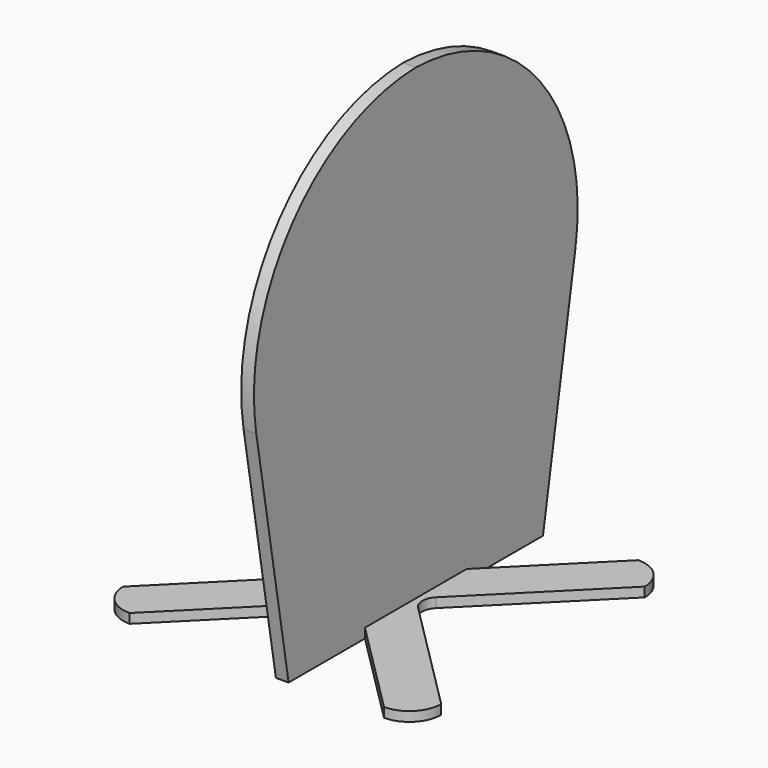
from build123d import *

# Parameters (mm, degrees)
F1_DEPTH    = 3
F2_R        = 9.99999
F3_R        = 5
F4_DEPTH    = 50
F6_DEPTH    = 10
F7_DEPTH    = 6
F8_T1_DEPTH = 387.2306894548
F9_R        = 9.99999
F10_R       = 5.99999


# Not quite as in the source:
# - a fillet or chamfer that OpenCascade refuses, or shapes differently, is made with other operations: its cross-section is extruded or revolved along the edge and cut away or added
# - a fillet or chamfer is up to 0.001 mm smaller than in the source, because OpenCascade refuses the exact size


with BuildPart() as f1:
    # F0 (on Top) → F1 (new body)
    with BuildSketch(Plane.XY):
        with BuildLine():
            Line((0, 10), (10, 0))
            ThreePointArc((10, 0), (7.0710678119, 7.0710678119), (0, 10))
        make_face()
        with BuildLine():
            Line((50, -40), (10, 0))
            ThreePointArc((10, 0), (7.0710678119, -7.0710678119), (0, -10))
            Line((0, -10), (40, -50))
            Line((40, -50), (50, -50))
            Line((50, -50), (50, -40))
        make_face()
        Polygon((0, -10), (10, 0), (0, 10), (-10, 0), align=None)
        with BuildLine():
            ThreePointArc((0, 10), (7.0710678119, 7.0710678119), (10, 0))
            Line((10, 0), (50, 40))
            Line((50, 40), (50, 50))
            Line((50, 50), (40, 50))
            Line((40, 50), (0, 10))
        make_face()
        with BuildLine():
            ThreePointArc((0, -10), (7.0710678119, -7.0710678119), (10, 0))
            Line((10, 0), (0, -10))
        make_face()
        with BuildLine():
            Line((-10, 0), (0, 10))
            ThreePointArc((0, 10), (-7.0710678119, 7.0710678119), (-10, 0))
        make_face()
        with BuildLine():
            ThreePointArc((-10, 0), (-7.0710678119, 7.0710678119), (0, 10))
            Line((0, 10), (-40, 50))
            Line((-40, 50), (-50, 50))
            Line((-50, 50), (-50, 40))
            Line((-50, 40), (-10, 0))
        make_face()
        with BuildLine():
            Line((-40, -50), (0, -10))
            ThreePointArc((0, -10), (-7.0710678119, -7.0710678119), (-10, 0))
            Line((-10, 0), (-50, -40))
            Line((-50, -40), (-50, -50))
            Line((-50, -50), (-40, -50))
        make_face()
        with BuildLine():
            ThreePointArc((-10, 0), (-7.0710678119, -7.0710678119), (0, -10))
            Line((0, -10), (-10, 0))
        make_face()
    extrude(amount=F1_DEPTH)

    # F2 (radius 10 in the source; OpenCascade refuses exactly that, so slightly less here)
    f2_edges = [f1.edges().sort_by_distance(p)[0] for p in [
        (-50, 50, 1.5),
        (-50, -50, 1.5),
        (50, -50, 1.5),
        (50, 50, 1.5),
    ]]
    fillet(f2_edges, radius=F2_R)

    # F3
    f3_edges = [f1.edges().sort_by_distance(p)[0] for p in [
        (10, 0, 1.5),
        (0, 10, 1.5),
        (-10, 0, 1.5),
        (0, -10, 1.5),
    ]]
    fillet(f3_edges, radius=F3_R)

    # F0 (on Top) → F4 (join)
    with BuildSketch(Plane.XY):
        with BuildLine():
            Line((0, 10), (10, 0))
            ThreePointArc((10, 0), (7.0710678119, 7.0710678119), (0, 10))
        make_face()
        Polygon((0, -10), (10, 0), (0, 10), (-10, 0), align=None)
        with BuildLine():
            ThreePointArc((0, -10), (7.0710678119, -7.0710678119), (10, 0))
            Line((10, 0), (0, -10))
        make_face()
        with BuildLine():
            Line((-10, 0), (0, 10))
            ThreePointArc((0, 10), (-7.0710678119, 7.0710678119), (-10, 0))
        make_face()
        with BuildLine():
            ThreePointArc((-10, 0), (-7.0710678119, -7.0710678119), (0, -10))
            Line((0, -10), (-10, 0))
        make_face()
    extrude(amount=F4_DEPTH)

    # F5 (on Right) → F6 (join)
    with BuildSketch(Plane.YZ):
        with BuildLine():
            Line((-70.7106781187, 120.7106781187), (0, 150))
            ThreePointArc((0, 150), (-37.3285426078, 146.4855717522), (-73.3452003698, 136.0657990677))
            Line((-73.3452003698, 136.0657990677), (-70.7106781187, 120.7106781187))
        make_face()
        Polygon((-64.6446609407, 85.3553390593), (0, 150), (-70.7106781187, 120.7106781187), align=None)
        Polygon((-50, 0), (0, 0), (0, 150), (-64.6446609407, 85.3553390593), align=None)
        Polygon((0, 150), (0, 0), (50, 0), (64.6446609407, 85.3553390593), align=None)
        Polygon((70.7106781187, 120.7106781187), (0, 150), (64.6446609407, 85.3553390593), align=None)
        with BuildLine():
            ThreePointArc((73.3452003698, 136.0657990677), (37.3285426078, 146.4855717522), (0, 150))
            Line((0, 150), (70.7106781187, 120.7106781187))
            Line((70.7106781187, 120.7106781187), (73.3452003698, 136.0657990677))
        make_face()
    extrude(amount=F6_DEPTH)

    # F7 (cut): a face of the model
    f7_faces = [f1.faces().sort_by_distance(p)[0] for p in [
        (0, 0, 80.6875743248),
    ]]
    extrude(f7_faces, amount=-F7_DEPTH, mode=Mode.SUBTRACT)

    # F8: fillet of radius 65 on 2 edges, made by hand

    # F8_s2 → F8_t1 (cut)
    with BuildSketch(Plane.YZ.offset(-185.6153447274)):
        with BuildLine():
            ThreePointArc((-62.6966411117, 74.0014474486), (-48.1162932181, 127.140168964), (2.0255781715, 149.9897423196))
            ThreePointArc((2.0255781715, 149.9897423196), (-36.3330590034, 146.6720845048), (-73.3452003698, 136.0657990677))
            Line((-73.3452003698, 136.0657990677), (-62.6966411117, 74.0014474486))
        make_face()
        with BuildLine():
            ThreePointArc((62.6966411117, 74.0014474486), (48.1162932181, 127.140168964), (-2.0255781715, 149.9897423196))
            ThreePointArc((-2.0255781715, 149.9897423196), (36.3330590034, 146.6720845048), (73.3452003698, 136.0657990677))
            Line((73.3452003698, 136.0657990677), (62.6966411117, 74.0014474486))
        make_face()
    extrude(amount=F8_T1_DEPTH, mode=Mode.SUBTRACT)

    # F9 (radius 10 in the source; OpenCascade refuses exactly that, so slightly less here)
    f9_edges = [f1.edges().sort_by_distance(p)[0] for p in [
        (-10, 0, 50),
        (3, 10, 50),
        (3, -10, 50),
    ]]
    fillet(f9_edges, radius=F9_R)

    # F10 (radius 6 in the source; OpenCascade refuses exactly that, so slightly less here)
    f10_edges = [f1.edges().sort_by_distance(p)[0] for p in [
        (6, 12.071068, 1.5),
        (6, -12.071068, 1.5),
    ]]
    fillet(f10_edges, radius=F10_R)


solid = f1.part
